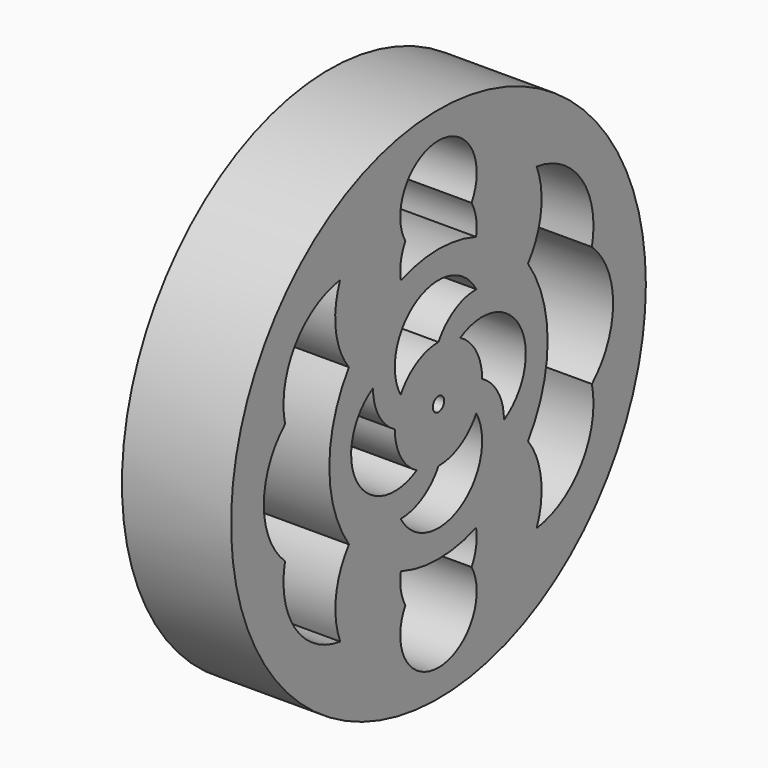
from build123d import *

# Parameters (mm, degrees)
F0_R     = 60.325
F0_R_2   = 1.651
F1_DEPTH = 25.4


# Not quite as in the source:
# - a feature names something its author has since deleted; it is built from what else it names


with BuildPart() as f1:
    # F0 (on Right) → F1 (new body)
    with BuildSketch(Plane.YZ):
        Circle(F0_R)
        with BuildLine():
            ThreePointArc((-44.6303828389, -14.0356060761), (-50.8, 0), (-44.6303828389, 14.0356060761))
            ThreePointArc((-44.6303828389, 14.0356060761), (-41.6692499302, 29.0570596505), (-28.609366898, 37.0477937078))
            ThreePointArc((-28.609366898, 37.0477937078), (-29.8846813864, 27.2910481481), (-26.1212663508, 18.1994466264))
            ThreePointArc((-26.1212663508, 18.1994466264), (-26.0781172223, 18.1860453578), (-26.035, 18.172541787))
            ThreePointArc((-26.035, 18.172541787), (-26.0505815045, 18.1501984364), (-26.0661438338, 18.1278417259))
            ThreePointArc((-26.0661438338, 18.1278417259), (-31.7499883148, -0.0272398323), (-26.035, -18.172541787))
            ThreePointArc((-26.035, -18.172541787), (-29.828858254, -27.2745235138), (-28.5634450169, -37.054000041))
            ThreePointArc((-28.5634450169, -37.054000041), (-41.656, -29.0760668592), (-44.6303828389, -14.0356060761))
        make_face(mode=Mode.SUBTRACT)
        with BuildLine():
            ThreePointArc((-19.05, 10.9985226281), (-17.3485226281, 4.6485226281), (-12.7, 0))
            ThreePointArc((-12.7, 0), (-10.9985226281, -6.35), (-6.35, -10.9985226281))
            ThreePointArc((-6.35, -10.9985226281), (-19.05, -10.9985226281), (-25.4, 0))
            ThreePointArc((-25.4, 0), (-25.3963047456, 0.4332496584), (-25.3852200578, 0.8663732563))
            ThreePointArc((-25.3852200578, 0.8663732563), (-25.3778345329, 0.8661197613), (-25.3704491069, 0.8658634012))
            ThreePointArc((-25.3704491069, 0.8658634012), (-23.4755309293, 6.7214532053), (-19.05, 10.9985226281))
        make_face(mode=Mode.SUBTRACT)
        with BuildLine():
            ThreePointArc((-9.6295053729, -37.3095975192), (-10.9516952283, -33.6727246106), (-10.9474, -29.8029685307))
            ThreePointArc((-10.9474, -29.8029685307), (0, -31.75), (10.9474, -29.8029685307))
            ThreePointArc((10.9474, -29.8029685307), (10.9516952283, -33.6727246106), (9.6295053729, -37.3095975192))
            ThreePointArc((9.6295053729, -37.3095975192), (0, -53.9883900769), (-9.6295053729, -37.3095975192))
        make_face(mode=Mode.SUBTRACT)
        with BuildLine():
            ThreePointArc((10.9985226281, -6.35), (6.35, -23.6985226281), (-10.9985226281, -19.05))
            ThreePointArc((-10.9985226281, -19.05), (-4.6485226281, -17.3485226281), (0, -12.7))
            ThreePointArc((0, -12.7), (6.35, -10.9985226281), (10.9985226281, -6.35))
        make_face(mode=Mode.SUBTRACT)
        with BuildLine():
            ThreePointArc((-10.9985226281, 6.35), (-6.35, 23.6985226281), (10.9985226281, 19.05))
            ThreePointArc((10.9985226281, 19.05), (4.6485226281, 17.3485226281), (0, 12.7))
            ThreePointArc((0, 12.7), (-6.35, 10.9985226281), (-10.9985226281, 6.35))
        make_face(mode=Mode.SUBTRACT)
        Circle(F0_R_2, mode=Mode.SUBTRACT)
        with BuildLine():
            ThreePointArc((6.35, 10.9985226281), (23.6985226281, 6.35), (19.05, -10.9985226281))
            ThreePointArc((19.05, -10.9985226281), (17.3485226281, -4.6485226281), (12.7, 0))
            ThreePointArc((12.7, 0), (10.9985226281, 6.35), (6.35, 10.9985226281))
        make_face(mode=Mode.SUBTRACT)
        with BuildLine():
            ThreePointArc((28.5634450169, -37.054000041), (29.828858254, -27.2745235138), (26.035, -18.172541787))
            ThreePointArc((26.035, -18.172541787), (31.75, 0), (26.035, 18.172541787))
            ThreePointArc((26.035, 18.172541787), (29.828858254, 27.2745235138), (28.5634450169, 37.054000041))
            ThreePointArc((28.5634450169, 37.054000041), (41.656, 29.0760668592), (44.6303828389, 14.0356060761))
            ThreePointArc((44.6303828389, 14.0356060761), (50.8, 0), (44.6303828389, -14.0356060761))
            ThreePointArc((44.6303828389, -14.0356060761), (41.656, -29.0760668592), (28.5634450169, -37.054000041))
        make_face(mode=Mode.SUBTRACT)
        with BuildLine():
            ThreePointArc((9.6295053729, 37.3095975192), (10.9516952283, 33.6727246106), (10.9474, 29.8029685307))
            ThreePointArc((10.9474, 29.8029685307), (0, 31.75), (-10.9474, 29.8029685307))
            ThreePointArc((-10.9474, 29.8029685307), (-10.9516952283, 33.6727246106), (-9.6295053729, 37.3095975192))
            ThreePointArc((-9.6295053729, 37.3095975192), (0, 53.9883900769), (9.6295053729, 37.3095975192))
        make_face(mode=Mode.SUBTRACT)
    extrude(amount=F1_DEPTH)


solid = f1.part
